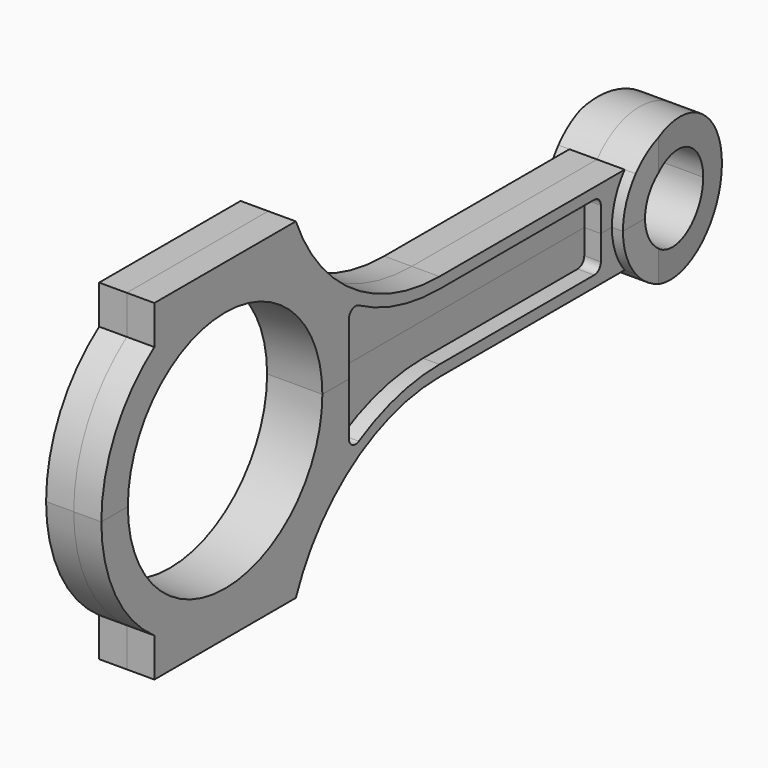
from build123d import *
from build123d import SkipClean  # not in build123d's __all__

# Parameters (mm, degrees)
F1_DEPTH = 7
F2_DEPTH = 5
F3_DEPTH = 2
F7_DEPTH = 25


with BuildPart() as f1:
    # F0 (on Right) → F1 (new body)
    with BuildSketch(Plane.YZ):
        with BuildLine():
            ThreePointArc((107.5, 0), (100, -7.5), (92.5, 0))
            Line((92.5, 0), (87.5, 0))
            ThreePointArc((87.5, 0), (88.2460947032, -4.2539052968), (90.3953136439, -8))
            ThreePointArc((90.3953136439, -8), (104.2539052968, -11.7539052968), (112.5, 0))
            Line((112.5, 0), (107.5, 0))
        make_face()
    extrude(amount=F1_DEPTH)

    # F0 (on Right) → F2 (join)
    with BuildSketch(Plane.YZ):
        with BuildLine():
            ThreePointArc((90.3953136439, -8), (88.2460947032, -4.2539052968), (87.5, 0))
            Line((87.5, 0), (85, 0))
            Line((85, 0), (85, -4.5))
            ThreePointArc((85, -4.5), (84.5606601718, -5.5606601718), (83.5, -6))
            Line((83.5, -6), (48.4961536185, -6))
            ThreePointArc((48.4961536185, -6), (39.0556702336, -7.2246275567), (30.2401098812, -10.8174446779))
            ThreePointArc((30.2401098812, -10.8174446779), (28.7450711364, -10.8089264191), (28, -9.5127464891))
            Line((28, -9.5127464891), (28, 0))
            Line((28, 0), (22, 0))
            ThreePointArc((22, 0), (0, -22), (-22, 0))
            Line((-22, 0), (-28, 0))
            ThreePointArc((-28, 0), (-24.819347292, -12.9614813968), (-16, -22.9782505862))
            Line((-16, -22.9782505862), (-16, -30))
            Line((-16, -30), (16, -30))
            ThreePointArc((16, -30), (28.8747367482, -14.0172465076), (48.4961536185, -8))
            Line((48.4961536185, -8), (90.3953136439, -8))
        make_face()
    extrude(amount=F2_DEPTH)

    # F0 (on Right) → F3 (join)
    with BuildSketch(Plane.YZ):
        with BuildLine():
            Line((85, -4.5), (85, 0))
            Line((85, 0), (28, 0))
            Line((28, 0), (28, -9.5127464891))
            ThreePointArc((28, -9.5127464891), (28.7450711364, -10.8089264191), (30.2401098812, -10.8174446779))
            ThreePointArc((30.2401098812, -10.8174446779), (39.0556702336, -7.2246275567), (48.4961536185, -6))
            Line((48.4961536185, -6), (83.5, -6))
            ThreePointArc((83.5, -6), (84.5606601718, -5.5606601718), (85, -4.5))
        make_face()
    extrude(amount=F3_DEPTH)

    # F4: F1 across plane


with BuildPart() as f1_1:
    add(f1.part, clean=False)
    add(f1.part.mirror(Plane.YZ), clean=False)

    # F5: F1 across plane


with BuildPart() as f1_2:
    add(f1_1.part, clean=False)
    with SkipClean():  # cleaning this boolean's faces spoils the solid; the shape is the same uncleaned
        add(f1_1.part.mirror(Plane.XY), clean=False)

    # F6 (on Top) → F7 (cut, symmetric)
    with BuildSketch(Plane.XY):
        Polygon((-7, 112.5), (-7, 95.5), (-4.9126624647, 112.5), align=None)
        Polygon((4.9126624647, 112.5), (7, 95.5), (7, 112.5), align=None)
    with SkipClean():  # cleaning this boolean's faces spoils the solid; the shape is the same uncleaned
        extrude(amount=F7_DEPTH, both=True, mode=Mode.SUBTRACT)


solid = f1_2.part
